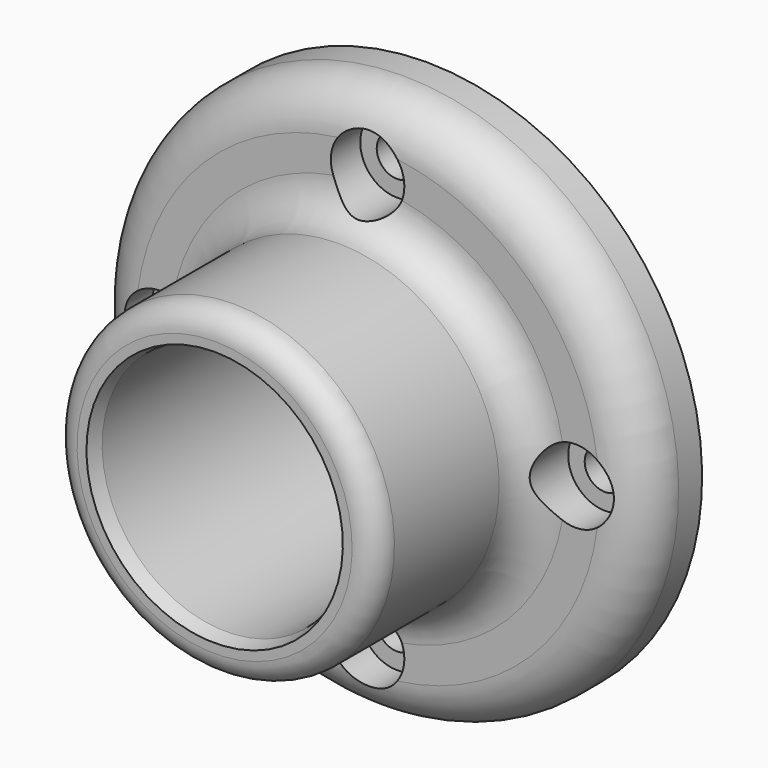
from build123d import *

# Parameters (mm, degrees)
F2_R           = 2.032
F4_D           = 3.5
F4_CBORE_D     = 6.35
F4_CBORE_DEPTH = 19.685


# Not quite as in the source:
# - a fillet or chamfer that OpenCascade refuses, or shapes differently, is made with other operations: its cross-section is extruded or revolved along the edge and cut away or added


with BuildPart() as f1:
    # F0 (on Right) → F1 (revolve)
    with BuildSketch(Plane.YZ):
        with BuildLine():
            Line((-22.86, 11.0717954744), (-21.59, 10.7315))
            Line((-21.59, 10.7315), (0, 10.7315))
            Line((0, 10.7315), (0, 23.8125))
            Line((0, 23.8125), (-6.35, 23.8125))
            Line((-6.35, 23.8125), (-6.35, 17.0815))
            ThreePointArc((-6.35, 17.0815), (-7.2799359697, 14.8364359697), (-9.525, 13.9065))
            Line((-9.525, 13.9065), (-22.86, 13.9065))
            Line((-22.86, 13.9065), (-22.86, 11.0717954744))
        make_face()
    revolve(axis=Axis((0, -11.43, 0), (0, -1, 0)))

    # F2
    f2_edges = [f1.edges().sort_by_distance(p)[0] for p in [
        (0, -22.86, -13.9065),
    ]]
    fillet(f2_edges, radius=F2_R)

    # F4 (through all)
    with Locations(Plane.XZ.offset(22.86)):
        with Locations((-17.9605122421, 0), (0, 17.9605122421), (17.9605122421, 0), (0, -17.9605122421)):
            CounterBoreHole(F4_D / 2, F4_CBORE_D / 2, F4_CBORE_DEPTH)

    # F5: fillet of radius 3.81 on 1 edges, made by hand

    # F5_s1 → F5_t2 (revolve, cut)
    with BuildSketch(Plane.YZ):
        with BuildLine():
            ThreePointArc((-6.35, 20.0025), (-5.2340768363, 22.6965768363), (-2.54, 23.8125))
            Line((-2.54, 23.8125), (-6.35, 23.8125))
            Line((-6.35, 23.8125), (-6.35, 20.0025))
        make_face()
    revolve(axis=Axis((0, -6.35, 0), (0, -1, 0)), mode=Mode.SUBTRACT)


solid = f1.part
